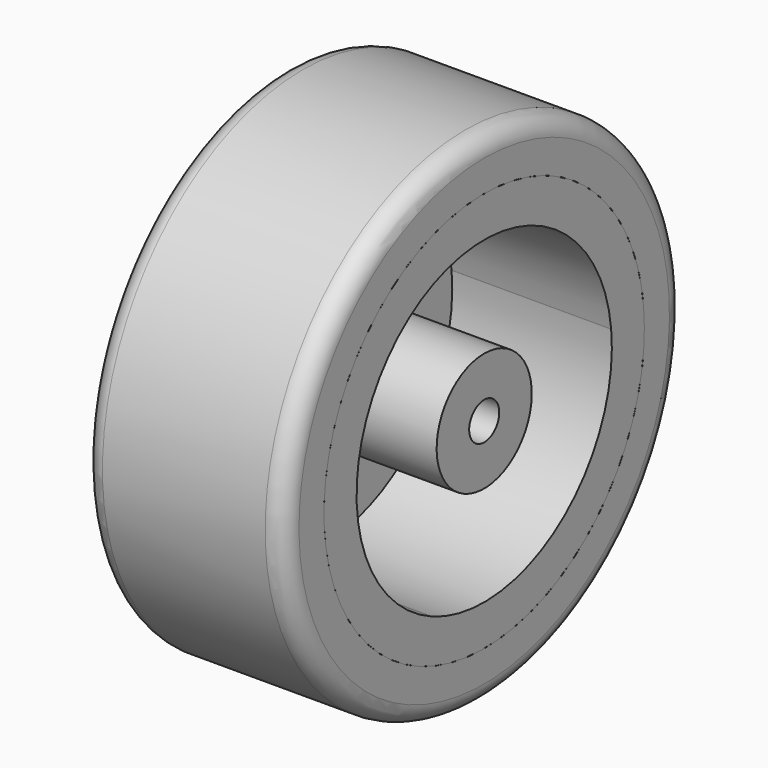
from build123d import *

# Parameters (mm, degrees)
F0_W      = 4
F0_H      = 1.5
F0_W_2    = 6
F0_H_2    = 2.5
F3_DEPTH  = 4
F4_R      = 1.5666851265
F5_DEPTH  = 1
F3_FACE_W = 4
F3_FACE_H = 10.6617561789
F7_DEPTH  = 6
F8_DEPTH  = 6
F9_T      = -3.25


with BuildPart() as f1:
    # F0 (on Front) → F1 (revolve)
    with BuildSketch(Plane.XZ):
        with BuildLine():
            Line((0, 2.5), (0, 0))
            Line((0, 0), (6, 0))
            Line((6, 0), (10, 0))
            Line((10, 0), (16, 0))
            Line((16, 0), (16, 2.5))
            ThreePointArc((16, 2.5), (15.5606601718, 3.5606601718), (14.5, 4))
            Line((14.5, 4), (1.5, 4))
            ThreePointArc((1.5, 4), (0.4393398282, 3.5606601718), (0, 2.5))
        make_face()
    revolve(axis=Axis((8, 0, -16), (1, 0, 0)))


with BuildPart() as f1b:
    # F0 (on Front) → F1, piece 2 (revolve)
    with BuildSketch(Plane.XZ):
        with Locations((8, -13.75)):
            Rectangle(F0_W, F0_H)
        with Locations((3, -13.75)):
            Rectangle(F0_W_2, F0_H)
        with Locations((8, -11.75)):
            Rectangle(F0_W, F0_H_2)
        with Locations((13, -13.75)):
            Rectangle(F0_W_2, F0_H)
    revolve(axis=Axis((8, 0, -16), (1, 0, 0)))

    # F2 (on face) → F3 (join)
    with BuildSketch(Plane(origin=(6, 0, 0), x_dir=(0, -1, 0), z_dir=(-1, 0, 0))):
        with BuildLine():
            Line((6.6908253366, -1.4861596642), (1.3844372123, -10.6770935002))
            ThreePointArc((1.3844372123, -10.6770935002), (2.8339033039, -11.2862974145), (4.051778006, -12.2807131073))
            Line((4.051778006, -12.2807131073), (9.3857185908, -3.0420570099))
            Line((9.3857185908, -3.0420570099), (6.6908253366, -1.4861596642))
        make_face()
        with BuildLine():
            ThreePointArc((4.037854872, -19.7343979479), (2.741097896, -20.7682682731), (1.1951079301, -21.36858613))
            Line((1.1951079301, -21.36858613), (6.5290485149, -30.6072422274))
            Line((6.5290485149, -30.6072422274), (9.3687329614, -28.9677496478))
            Line((9.3687329614, -28.9677496478), (4.037854872, -19.7343979479))
        make_face()
        with BuildLine():
            ThreePointArc((-5.3019908569, -17.4624954541), (-5.4991378368, -15.9026190397), (-5.246885936, -14.3507007627))
            Line((-5.246885936, -14.3507007627), (-15.9147671056, -14.3507007627))
            Line((-15.9147671056, -14.3507007627), (-15.9147671056, -17.4624954541))
            Line((-15.9147671056, -17.4624954541), (-5.3019908569, -17.4624954541))
        make_face()
    extrude(amount=-F3_DEPTH)

    # F4 (on Right) → F5 (join)
    with BuildSketch(Plane.YZ):
        with Locations((0, -15.8851090819)):
            Circle(F4_R)
    extrude(amount=F5_DEPTH)

    # F3_face (on face) → F6 (revolve)
    with BuildSketch(Plane(origin=(8, -6.7032939167, -24.3510737978), x_dir=(1, 0, 0), z_dir=(0, -0.8660254038, 0.5))):
        Rectangle(F3_FACE_W, F3_FACE_H)
    revolve(axis=Axis((16, 0, -16), (1, 0, 0)))

    # F7 (add): a face of the model
    f7_faces = [f1b.faces().sort_by_distance(p)[0] for p in [
        (10, 6.3521420728, -1.8115251344),
    ]]
    extrude(f7_faces, amount=F7_DEPTH)

    # F8 (add): a face of the model
    f8_faces = [f1b.faces().sort_by_distance(p)[0] for p in [
        (6, 0, -19.4524914923),
    ]]
    extrude(f8_faces, amount=F8_DEPTH)

    # F9
    f9_openings = [f1b.faces().sort_by_distance(p)[0] for p in [
        (16, 0, -17.952491),
    ]]
    offset(amount=F9_T, openings=f9_openings)


solid = Compound([f1.part, f1b.part])
